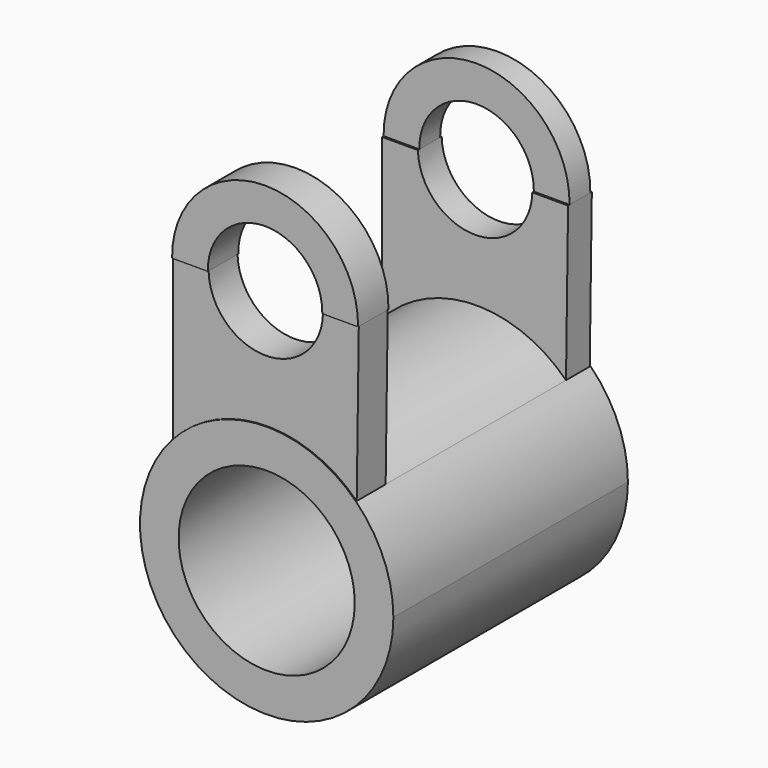
from build123d import *

# Parameters (mm, degrees)
F0_R     = 24.113842
F1_DEPTH = 40.132
F2_START = -31.75
F2_DEPTH = 8.128
F3_START = 29.972
F3_DEPTH = 9.906
F4_START = 29.718
F4_DEPTH = 10.414
F5_START = -32.258
F5_DEPTH = 7.112


with BuildPart() as f1:
    # F0 (on Front) → F1 (new body, symmetric)
    with BuildSketch(Plane.XZ):
        with BuildLine():
            ThreePointArc((-25.896491, 23.080411), (-12.349244, -32.416505), (34.6891, 0))
            ThreePointArc((34.6891, 0), (32.02648, 13.328099), (24.447368, 24.610157))
            ThreePointArc((24.447368, 24.610157), (-1.053575, 34.673096), (-25.896491, 23.080411))
        make_face()
        Circle(F0_R, mode=Mode.SUBTRACT)
    extrude(amount=F1_DEPTH, both=True)

    # F0 (on Front) → F2 (join)
    with BuildSketch(Plane.XZ.offset(F2_START)):
        with BuildLine():
            ThreePointArc((-25.896491, 23.080411), (-1.053575, 34.673096), (24.447368, 24.610157))
            Line((24.447368, 24.610157), (25.016466, 66.879792))
            Line((25.016466, 66.879792), (15.218874, 66.879792))
            ThreePointArc((15.218874, 66.879792), (-0.440013, 51.559889), (-16.0989, 66.879792))
            Line((-16.0989, 66.879792), (-25.896491, 66.879792))
            Line((-25.896491, 66.879792), (-25.896491, 23.080411))
        make_face()
    extrude(amount=-F2_DEPTH)

    # F0 (on Front) → F3 (join)
    with BuildSketch(Plane.XZ.offset(F3_START)):
        with BuildLine():
            ThreePointArc((-25.896491, 23.080411), (-1.053575, 34.673096), (24.447368, 24.610157))
            Line((24.447368, 24.610157), (25.016466, 66.879792))
            Line((25.016466, 66.879792), (15.218874, 66.879792))
            ThreePointArc((15.218874, 66.879792), (-0.440013, 51.559889), (-16.0989, 66.879792))
            Line((-16.0989, 66.879792), (-25.896491, 66.879792))
            Line((-25.896491, 66.879792), (-25.896491, 23.080411))
        make_face()
    extrude(amount=F3_DEPTH)

    # F0 (on Front) → F4 (join)
    with BuildSketch(Plane.XZ.offset(F4_START)):
        with BuildLine():
            Line((15.218874, 66.879792), (25.016466, 66.879792))
            ThreePointArc((25.016466, 66.879792), (-0.440013, 92.681312), (-25.896491, 66.879792))
            Line((-25.896491, 66.879792), (-16.0989, 66.879792))
            ThreePointArc((-16.0989, 66.879792), (-0.61139, 82.884226), (15.222625, 67.222526))
            ThreePointArc((15.222625, 67.222526), (15.221687, 67.051149), (15.218874, 66.879792))
        make_face()
    extrude(amount=F4_DEPTH)

    # F0 (on Front) → F5 (join)
    with BuildSketch(Plane.XZ.offset(F5_START)):
        with BuildLine():
            Line((15.218874, 66.879792), (25.016466, 66.879792))
            ThreePointArc((25.016466, 66.879792), (-0.440013, 92.681312), (-25.896491, 66.879792))
            Line((-25.896491, 66.879792), (-16.0989, 66.879792))
            ThreePointArc((-16.0989, 66.879792), (-0.61139, 82.884226), (15.222625, 67.222526))
            ThreePointArc((15.222625, 67.222526), (15.221687, 67.051149), (15.218874, 66.879792))
        make_face()
    extrude(amount=-F5_DEPTH)


solid = f1.part
